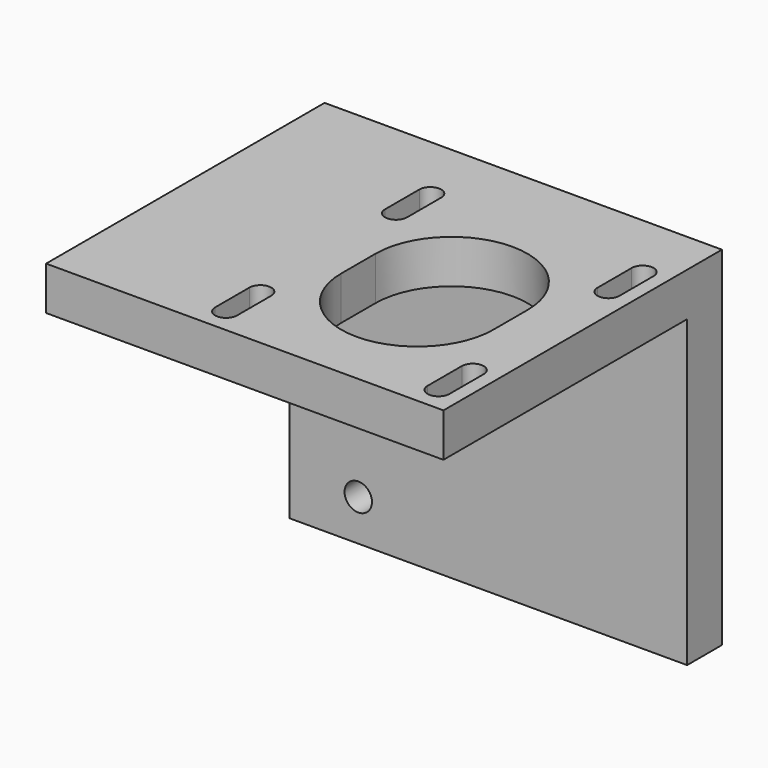
from build123d import *

# Parameters (mm, degrees)
F0_W     = 57.99
F0_H     = 6.35
F0_H_2   = 44.45
F1_DEPTH = 6.35
F2_DEPTH = 44.45
F3_R     = 2
F4_DEPTH = 50.801


# Not quite as in the source:
# - a length typed as a fraction of an inch, garbled in the dataset ("3 / 203.2 mm" for 3/8 in), is restored
# - a feature names something its author has since deleted; it is built from what else it names


with BuildPart() as f1:
    # F0 (on Top) → F1 (new body)
    with BuildSketch(Plane.XY):
        with Locations((-9.895, 22.275)):
            Rectangle(F0_W, F0_H)
        with Locations((-9.895, -3.125)):
            Rectangle(F0_W, F0_H_2)
        with BuildLine():
            ThreePointArc((-17.1, -15.5), (-15.5, -13.9), (-13.9, -15.5))
            Line((-13.9, -15.5), (-13.9, -21.75))
            ThreePointArc((-13.9, -21.75), (-15.5, -23.35), (-17.1, -21.75))
            Line((-17.1, -21.75), (-17.1, -15.5))
        make_face(mode=Mode.SUBTRACT)
        with BuildLine():
            ThreePointArc((13.9, -15.5), (15.5, -13.9), (17.1, -15.5))
            Line((17.1, -15.5), (17.1, -21.75))
            ThreePointArc((17.1, -21.75), (15.5, -23.35), (13.9, -21.75))
            Line((13.9, -21.75), (13.9, -15.5))
        make_face(mode=Mode.SUBTRACT)
        with BuildLine():
            ThreePointArc((-11.1, 0), (0, 11.1), (11.1, 0))
            Line((11.1, 0), (11.1, -6.25))
            ThreePointArc((11.1, -6.25), (0, -17.35), (-11.1, -6.25))
            Line((-11.1, -6.25), (-11.1, 0))
        make_face(mode=Mode.SUBTRACT)
        with BuildLine():
            ThreePointArc((-17.1, 15.5), (-15.5, 17.1), (-13.9, 15.5))
            Line((-13.9, 15.5), (-13.9, 9.25))
            ThreePointArc((-13.9, 9.25), (-15.5, 7.65), (-17.1, 9.25))
            Line((-17.1, 9.25), (-17.1, 15.5))
        make_face(mode=Mode.SUBTRACT)
        with BuildLine():
            ThreePointArc((13.9, 15.5), (15.5, 17.1), (17.1, 15.5))
            Line((17.1, 15.5), (17.1, 9.25))
            ThreePointArc((17.1, 9.25), (15.5, 7.65), (13.9, 9.25))
            Line((13.9, 9.25), (13.9, 15.5))
        make_face(mode=Mode.SUBTRACT)
    extrude(amount=F1_DEPTH)

    # F0 (on Top) → F2 (join)
    with BuildSketch(Plane.XY):
        with Locations((-9.895, 22.275)):
            Rectangle(F0_W, F0_H)
    extrude(amount=-F2_DEPTH)

    # F3 (on face) → F4 (cut, through all)
    with BuildSketch(Plane(origin=(0, 25.45, 0), x_dir=(-1, 0, 0), z_dir=(0, 1, 0))):
        with Locations((28.89, -6)):
            Circle(F3_R)
        with Locations((28.89, -38.45)):
            Circle(F3_R)
    extrude(amount=-F4_DEPTH, mode=Mode.SUBTRACT)


solid = f1.part
